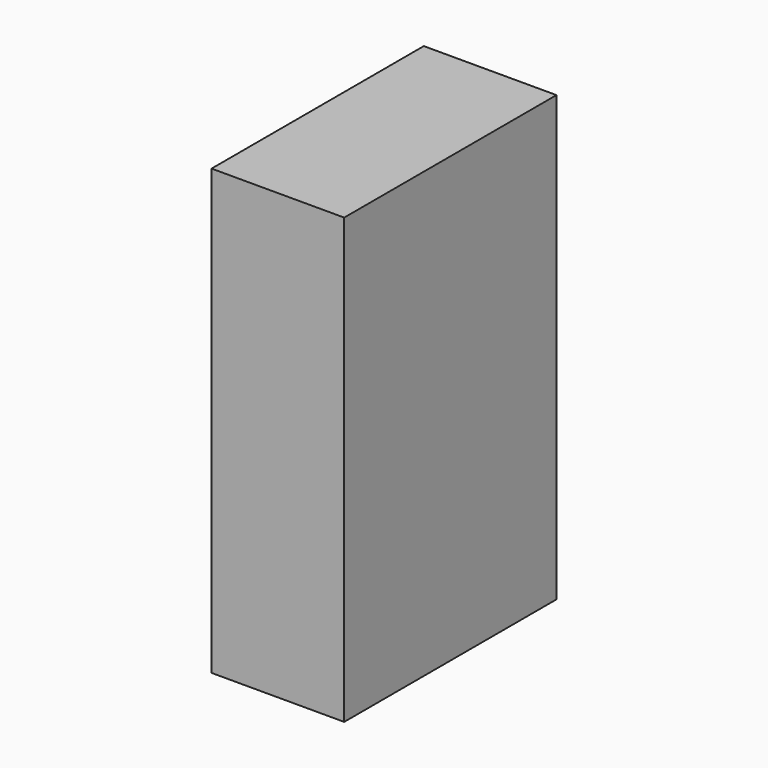
from build123d import *

# Parameters (mm, degrees)
F1_E0_RIGHT_W = 85.0174725056
F1_E0_RIGHT_H = 25.4
F2_DEPTH      = 50.8


with BuildPart() as f2:
    # F1_E0_right (on explicit) → F2 (new body)
    with BuildSketch(Plane(origin=(0, -39.9113744497, 0), x_dir=(0, 0, -1), z_dir=(0, -1, 0))):
        with Locations((42.5087362528, 12.7)):
            Rectangle(F1_E0_RIGHT_W, F1_E0_RIGHT_H)
    extrude(amount=F2_DEPTH)


solid = f2.part
